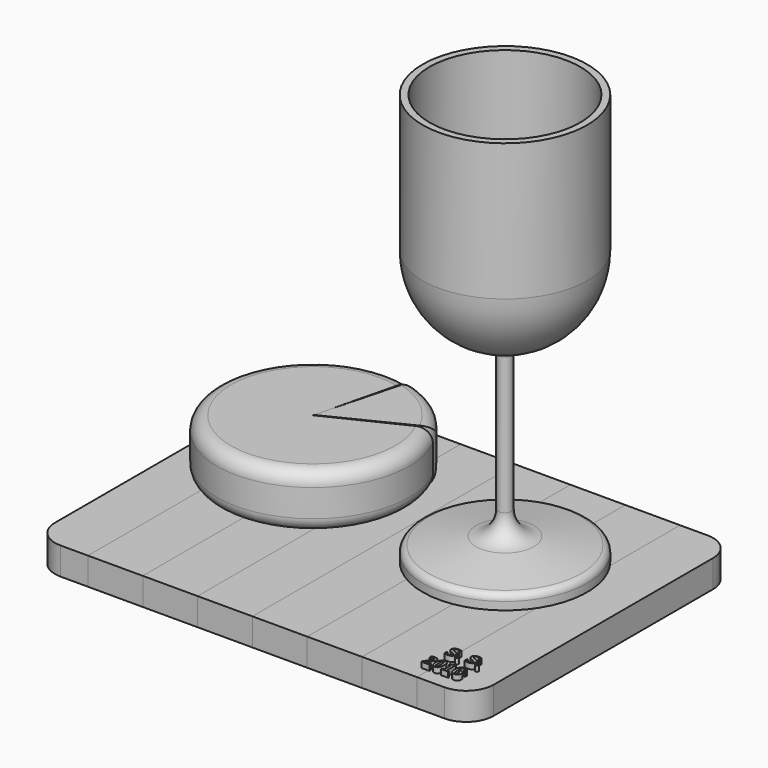
from build123d import *

# Parameters (mm, degrees)
F5_DEPTH      = 12.7
F4_W          = 25.4
F4_H          = 152.4
F6_DEPTH      = 12.7
F7_R          = 44.45
F8_DEPTH      = 25.4
F9_R          = 6.35
F11_DEPTH     = 25.4
F13_DEPTH     = 25.4
F14_R         = 5.08
F15_TEXT_SIZE = 8.8194630882
F16_DEPTH     = 2.54


# Not quite as in the source:
# - Text() gives the source's letters only with a copy of the font that has no kerning and outlines rounded to 1/6400 em; it was checked with that copy


with BuildPart() as f1:
    # F0 (on Front) → F1 (revolve)
    with BuildSketch(Plane.XZ):
        with BuildLine():
            Line((-38.1, 0), (0, 0))
            Line((0, 0), (0, 12.7))
            Line((0, 12.7), (0, 88.9))
            Line((0, 88.9), (0, 92.075))
            ThreePointArc((0, 92.075), (-24.6957043329, 102.3042956671), (-34.925, 127))
            Line((-34.925, 127), (-34.925, 190.5))
            Line((-34.925, 190.5), (-38.1, 190.5))
            Line((-38.1, 190.5), (-38.1, 127))
            ThreePointArc((-38.1, 127), (-29.1428063615, 102.4580596248), (-6.4828431823, 89.4555897067))
            ThreePointArc((-6.4828431823, 89.4555897067), (-4.0953752309, 87.8289235499), (-3.175, 85.090501479))
            Line((-3.175, 85.090501479), (-3.175, 21.590501479))
            ThreePointArc((-3.175, 21.590501479), (-6.0981667353, 14.0614102957), (-13.3360178534, 10.4773303578))
            Line((-13.3360178534, 10.4773303578), (-35.4469667847, 6.7921722026))
            ThreePointArc((-35.4469667847, 6.7921722026), (-37.3475884444, 5.7126117896), (-38.1, 3.6603714944))
            Line((-38.1, 3.6603714944), (-38.1, 0))
        make_face()
    revolve(axis=Axis((0, 0, 97.183718419), (0, 0, -1)))


with BuildPart() as f3:
    # F2 (on Front) → F3 (revolve)
    with BuildSketch(Plane.XZ):
        with BuildLine():
            Line((0, 93.037083745), (0, 148.840883745))
            Line((0, 148.840883745), (-34.5668382943, 148.840883745))
            Line((-34.5668382943, 148.840883745), (-34.5668382943, 126.9857734442))
            ThreePointArc((-34.5668382943, 126.9857734442), (-24.4042981415, 102.760890359), (0, 93.037083745))
        make_face()
    revolve(axis=Axis((0, 0, 50.8), (0, 0, 1)))


with BuildPart() as f5:
    # F4 (on Top) → F5 (new body)
    with BuildSketch(Plane.XY):
        with BuildLine():
            Line((-120.8394557322, -90.443163394), (-120.8394557322, 61.956836606))
            Line((-120.8394557322, 61.956836606), (-133.5394557322, 61.956836606))
            ThreePointArc((-133.5394557322, 61.956836606), (-142.5197118533, 58.2370927271), (-146.2394557322, 49.256836606))
            Line((-146.2394557322, 49.256836606), (-146.2394557322, -77.743163394))
            ThreePointArc((-146.2394557322, -77.743163394), (-142.5197118533, -86.7234195151), (-133.5394557322, -90.443163394))
            Line((-133.5394557322, -90.443163394), (-120.8394557322, -90.443163394))
        make_face()
    extrude(amount=-F5_DEPTH)


with BuildPart() as f5b:
    # F4 (on Top) → F5, piece 2 (new body)
    with BuildSketch(Plane.XY):
        with Locations((-82.7394557322, -14.243163394)):
            Rectangle(F4_W, F4_H)
    extrude(amount=-F5_DEPTH)


with BuildPart() as f5c:
    # F4 (on Top) → F5, piece 3 (new body)
    with BuildSketch(Plane.XY):
        with Locations((-31.9394557322, -14.243163394)):
            Rectangle(F4_W, F4_H)
    extrude(amount=-F5_DEPTH)


with BuildPart() as f5d:
    # F4 (on Top) → F5, piece 4 (new body)
    with BuildSketch(Plane.XY):
        with Locations((18.8605442678, -14.243163394)):
            Rectangle(F4_W, F4_H)
    extrude(amount=-F5_DEPTH)


with BuildPart() as f6:
    # F4 (on Top) → F6 (new body)
    with BuildSketch(Plane.XY):
        with Locations((-108.1394557322, -14.243163394)):
            Rectangle(F4_W, F4_H)
    extrude(amount=-F6_DEPTH)


with BuildPart() as f6b:
    # F4 (on Top) → F6, piece 2 (new body)
    with BuildSketch(Plane.XY):
        with Locations((-57.3394557322, -14.243163394)):
            Rectangle(F4_W, F4_H)
    extrude(amount=-F6_DEPTH)


with BuildPart() as f6c:
    # F4 (on Top) → F6, piece 3 (new body)
    with BuildSketch(Plane.XY):
        with Locations((-6.5394557322, -14.243163394)):
            Rectangle(F4_W, F4_H)
    extrude(amount=-F6_DEPTH)


with BuildPart() as f6d:
    # F4 (on Top) → F6, piece 4 (new body)
    with BuildSketch(Plane.XY):
        with BuildLine():
            ThreePointArc((56.9605442678, 49.256836606), (53.2408003888, 58.2370927271), (44.2605442678, 61.956836606))
            Line((44.2605442678, 61.956836606), (31.5605442678, 61.956836606))
            Line((31.5605442678, 61.956836606), (31.5605442678, -90.443163394))
            Line((31.5605442678, -90.443163394), (44.2605442678, -90.443163394))
            ThreePointArc((44.2605442678, -90.443163394), (53.2408003888, -86.7234195151), (56.9605442678, -77.743163394))
            Line((56.9605442678, -77.743163394), (56.9605442678, 49.256836606))
        make_face()
    extrude(amount=-F6_DEPTH)

    # F15 (on face) → F16 (join)
    with BuildSketch(Plane.XY):
        with Locations(Location((30.1705246019, -73.6729332929), (0, 0, 0.1178102965))):
            Text('S. S.', F15_TEXT_SIZE, font='Tinos', font_style=FontStyle.BOLD, text_align=(TextAlign.LEFT, TextAlign.BOTTOM))
        with Locations(Location((27.9865180156, -83.8198279963), (0, 0, 0.1178102965))):
            Text('2016', F15_TEXT_SIZE, font='Tinos', font_style=FontStyle.BOLD, text_align=(TextAlign.LEFT, TextAlign.BOTTOM))
    extrude(amount=F16_DEPTH)


with BuildPart() as f8:
    # F7 (on face) → F8 (new body)
    with BuildSketch(Plane.XY):
        with Locations((-95.4394557322, 8.160546422)):
            Circle(F7_R)
    extrude(amount=F8_DEPTH)

    # F9
    f9_edges = [f8.edges().sort_by_distance(p)[0] for p in [
        (-139.889456, 8.160546, 25.4),
        (-50.989456, 8.160546, 12.7),
        (-139.889456, 8.160546, 0),
    ]]
    fillet(f9_edges, radius=F9_R)

    # F10 (on face) → F11 (cut)
    with BuildSketch(Plane.XY.offset(25.4)):
        with BuildLine():
            Line((-84.7581235543, 51.3081030493), (-95.4394557322, 8.160546422))
            Line((-95.4394557322, 8.160546422), (-55.4643075532, 27.5973678717))
            ThreePointArc((-55.4643075532, 27.5973678717), (-51.4722938034, 62.4804965199), (-84.7581235543, 51.3081030493))
        make_face()
    extrude(amount=-F11_DEPTH, mode=Mode.SUBTRACT)


with BuildPart() as f13:
    # F12 (on face) → F13 (new body)
    with BuildSketch(Plane.XY):
        with BuildLine():
            Line((-84.1211936447, 51.4387148104), (-95.4394557322, 8.5529815406))
            Line((-95.4394557322, 8.5529815406), (-55.6790304603, 28.2099842869))
            ThreePointArc((-55.6790304603, 28.2099842869), (-67.3832343897, 42.9061126751), (-84.1211936447, 51.4387148104))
        make_face()
    extrude(amount=F13_DEPTH)

    # F14
    f14_edges = [f13.edges().sort_by_distance(p)[0] for p in [
        (-55.67903, 28.209984, 12.7),
        (-84.121194, 51.438715, 12.7),
        (-67.383234, 42.906113, 0),
        (-67.383234, 42.906113, 25.4),
    ]]
    fillet(f14_edges, radius=F14_R)


solid = Compound([f1.part, f3.part, f5.part, f5b.part, f5c.part, f5d.part, f6.part, f6b.part, f6c.part, f6d.part, f8.part, f13.part])
